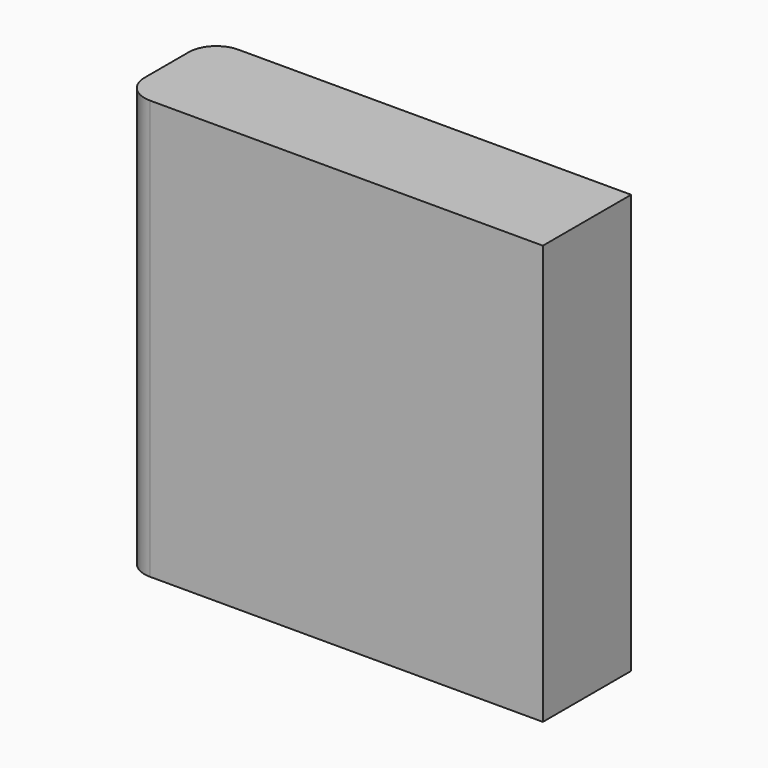
from build123d import *

# Parameters (mm, degrees)
F0_W     = 76.1904343963
F0_H     = 75.98939538
F1_DEPTH = 20
F4_R     = 5


# Not quite as in the source:
# - the program builds the solid bodies; features that only make, move or delete a surface that nothing else refers to are left out


with BuildPart() as f1:
    # F0 (on Front) → F1 (new body)
    with BuildSketch(Plane.XZ):
        with Locations((38.0952171981, 37.99469769)):
            Rectangle(F0_W, F0_H)
    extrude(amount=F1_DEPTH)

    # F4
    f4_edges = [f1.edges().sort_by_distance(p)[0] for p in [
        (0, -20, 37.994698),
        (0, 0, 37.994698),
    ]]
    fillet(f4_edges, radius=F4_R)


solid = f1.part
